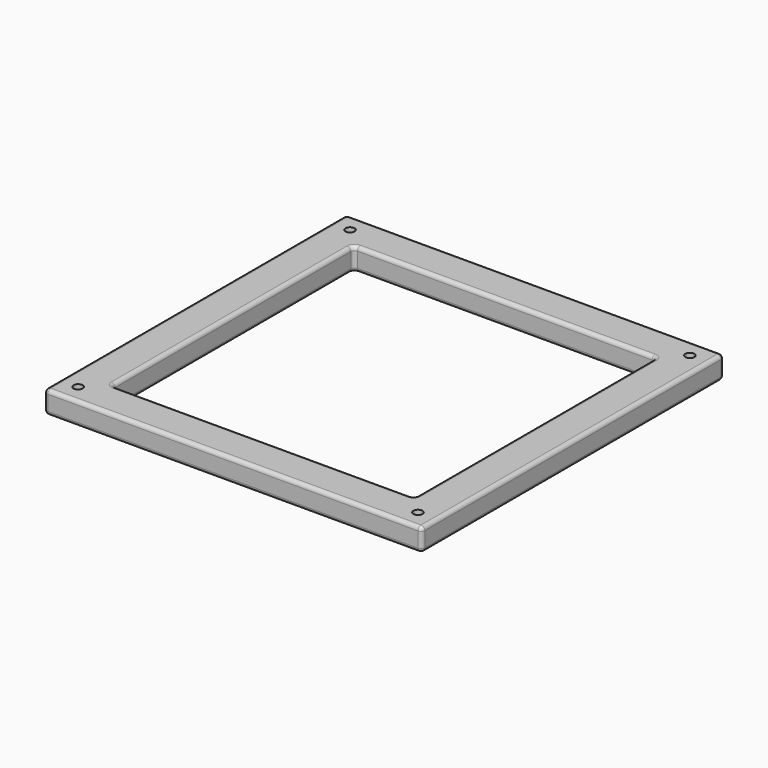
from build123d import *

# Parameters (mm, degrees)
F0_W     = 500
F0_H     = 500
F0_R     = 6
F0_W_2   = 400
F0_H_2   = 400
F1_DEPTH = 30
F6_F1_R  = 5
F6_F2_R  = 5
F6_F3_R  = 5


with BuildPart() as f1:
    # F0 (on Top) → F1 (new body)
    with BuildSketch(Plane.XY):
        Rectangle(F0_W, F0_H)
        with Locations((-225, -225)):
            Circle(F0_R, mode=Mode.SUBTRACT)
        with Locations((225, -225)):
            Circle(F0_R, mode=Mode.SUBTRACT)
        with Locations((-225, 225)):
            Circle(F0_R, mode=Mode.SUBTRACT)
        Rectangle(F0_W_2, F0_H_2, mode=Mode.SUBTRACT)
        with Locations((225, 225)):
            Circle(F0_R, mode=Mode.SUBTRACT)
    extrude(amount=F1_DEPTH)

    # F6: fillet of radius 5 on 22 edges, made by hand

    # F6_f1
    f6_f1_edges = [f1.edges().sort_by_distance(p)[0] for p in [
        (-200, -200, 15),
        (-200, 200, 15),
        (200, 200, 15),
        (200, -200, 15),
    ]]
    fillet(f6_f1_edges, radius=F6_F1_R)

    # F6_f2
    f6_f2_edges = [f1.edges().sort_by_distance(p)[0] for p in [
        (250, -250, 15),
        (250, 250, 15),
        (250, 0, 0),
        (250, 0, 30),
        (-250, 250, 15),
        (0, 250, 0),
        (0, 250, 30),
        (-250, 0, 30),
        (-250, -250, 15),
        (-250, 0, 0),
        (0, -250, 0),
        (0, -250, 30),
    ]]
    fillet(f6_f2_edges, radius=F6_F2_R)

    # F6_f3
    f6_f3_edges = [f1.edges().sort_by_distance(p)[0] for p in [
        (-200, 0, 0),
        (-200, 0, 30),
        (0, 200, 0),
        (0, 200, 30),
        (0, -200, 0),
        (0, -200, 30),
        (198.5355339059, -198.5355339059, 30),
        (-198.5355339059, -198.5355339059, 30),
        (198.5355339059, -198.5355339059, 0),
        (-198.5355339059, -198.5355339059, 0),
        (-198.5355339059, 198.5355339059, 30),
        (198.5355339059, 198.5355339059, 30),
        (-198.5355339059, 198.5355339059, 0),
        (198.5355339059, 198.5355339059, 0),
    ]]
    fillet(f6_f3_edges, radius=F6_F3_R)


solid = f1.part
